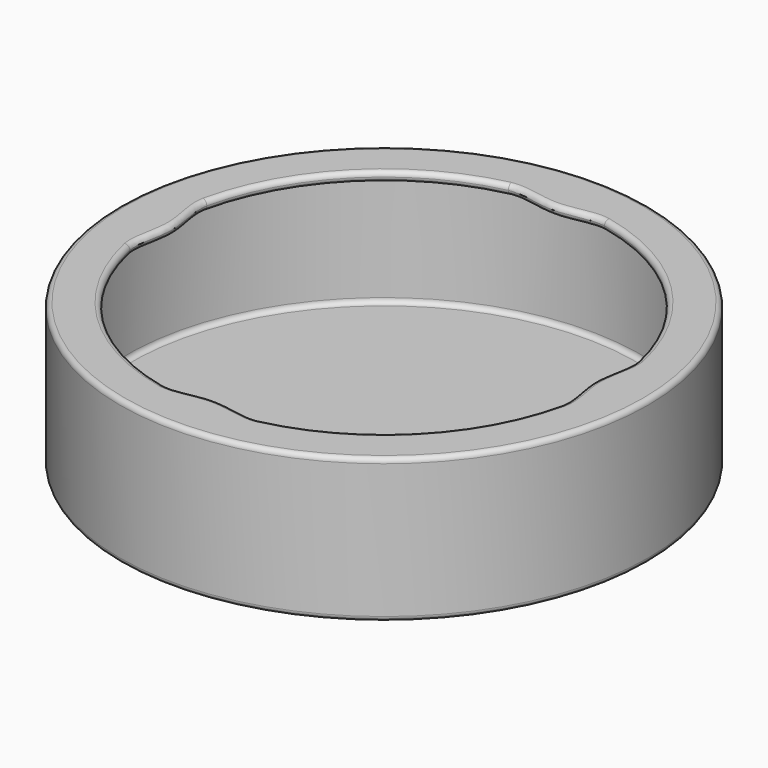
from build123d import *

# Parameters (mm, degrees)
F0_R     = 27.5
F0_R_2   = 26.75
F1_DEPTH = 1
F2_DEPTH = 15
F3_START = 14
F3_DEPTH = 1
F4_R     = 0.4999


# Not quite as in the source:
# - a fillet or chamfer is up to 0.001 mm smaller than in the source, because OpenCascade refuses the exact size


with BuildPart() as f1:
    # F0 (on Top) → F1 (new body)
    with BuildSketch(Plane.XY):
        Circle(F0_R)
        Circle(F0_R_2, mode=Mode.SUBTRACT)
        Circle(F0_R_2)
        with BuildLine():
            ThreePointArc((22.4499443206, 5), (22.8620725151, 2.5150825658), (23, 0))
            ThreePointArc((23, 0), (22.8620725151, -2.5150825658), (22.4499443206, -5))
            ThreePointArc((22.4499443206, -5), (16.2634559673, -16.2634559673), (5, -22.4499443206))
            ThreePointArc((5, -22.4499443206), (0, -23), (-5, -22.4499443206))
            ThreePointArc((-5, -22.4499443206), (-16.2634559673, -16.2634559673), (-22.4499443206, -5))
            ThreePointArc((-22.4499443206, -5), (-23, 0), (-22.4499443206, 5))
            ThreePointArc((-22.4499443206, 5), (-16.2634559673, 16.2634559673), (-5, 22.4499443206))
            ThreePointArc((-5, 22.4499443206), (0, 23), (5, 22.4499443206))
            ThreePointArc((5, 22.4499443206), (16.2634559673, 16.2634559673), (22.4499443206, 5))
        make_face(mode=Mode.SUBTRACT)
        with BuildLine():
            add(Edge.make_bspline(
                [(22.4499443206, 5), (22.7321358433, 3.5), (21.2678641567, 0), (22.7321358433, -3.5), (22.4499443206, -5)],
                knots=[0, 0, 0, 0, 0.5, 1, 1, 1, 1], degree=3))
            ThreePointArc((22.4499443206, 5), (16.2634559673, 16.2634559673), (5, 22.4499443206))
            add(Edge.make_bspline(
                [(-5, 22.4499443206), (-3.5, 22.7321358433), (0, 21.2678641567), (3.5, 22.7321358433), (5, 22.4499443206)],
                knots=[0, 0, 0, 0, 0.5, 1, 1, 1, 1], degree=3))
            ThreePointArc((-5, 22.4499443206), (-16.2634559673, 16.2634559673), (-22.4499443206, 5))
            add(Edge.make_bspline(
                [(-22.4499443206, 5), (-22.7321358433, 3.5), (-21.2678641567, 0), (-22.7321358433, -3.5), (-22.4499443206, -5)],
                knots=[0, 0, 0, 0, 0.5, 1, 1, 1, 1], degree=3))
            ThreePointArc((-22.4499443206, -5), (-16.2634559673, -16.2634559673), (-5, -22.4499443206))
            add(Edge.make_bspline(
                [(-5, -22.4499443206), (-3.5, -22.7321358433), (0, -21.2678641567), (3.5, -22.7321358433), (5, -22.4499443206)],
                knots=[0, 0, 0, 0, 0.5, 1, 1, 1, 1], degree=3))
            ThreePointArc((5, -22.4499443206), (16.2634559673, -16.2634559673), (22.4499443206, -5))
        make_face()
        with BuildLine():
            ThreePointArc((-5, -22.4499443206), (0, -23), (5, -22.4499443206))
            add(Edge.make_bspline(
                [(-5, -22.4499443206), (-3.5, -22.7321358433), (0, -21.2678641567), (3.5, -22.7321358433), (5, -22.4499443206)],
                knots=[0, 0, 0, 0, 0.5, 1, 1, 1, 1], degree=3))
        make_face()
        with BuildLine():
            add(Edge.make_bspline(
                [(-5, 22.4499443206), (-3.5, 22.7321358433), (0, 21.2678641567), (3.5, 22.7321358433), (5, 22.4499443206)],
                knots=[0, 0, 0, 0, 0.5, 1, 1, 1, 1], degree=3))
            ThreePointArc((5, 22.4499443206), (0, 23), (-5, 22.4499443206))
        make_face()
        with BuildLine():
            add(Edge.make_bspline(
                [(-22.4499443206, 5), (-22.7321358433, 3.5), (-21.2678641567, 0), (-22.7321358433, -3.5), (-22.4499443206, -5)],
                knots=[0, 0, 0, 0, 0.5, 1, 1, 1, 1], degree=3))
            ThreePointArc((-22.4499443206, 5), (-23, 0), (-22.4499443206, -5))
        make_face()
        with BuildLine():
            ThreePointArc((22.4499443206, -5), (22.8620725151, -2.5150825658), (23, 0))
            ThreePointArc((23, 0), (22.8620725151, 2.5150825658), (22.4499443206, 5))
            add(Edge.make_bspline(
                [(22.4499443206, 5), (22.7321358433, 3.5), (21.2678641567, 0), (22.7321358433, -3.5), (22.4499443206, -5)],
                knots=[0, 0, 0, 0, 0.5, 1, 1, 1, 1], degree=3))
        make_face()
    extrude(amount=F1_DEPTH)

    # F0 (on Top) → F2 (join)
    with BuildSketch(Plane.XY):
        Circle(F0_R)
        Circle(F0_R_2, mode=Mode.SUBTRACT)
    extrude(amount=F2_DEPTH)

    # F0 (on Top) → F3 (join)
    with BuildSketch(Plane.XY.offset(F3_START)):
        Circle(F0_R)
        Circle(F0_R_2, mode=Mode.SUBTRACT)
        Circle(F0_R_2)
        with BuildLine():
            ThreePointArc((22.4499443206, 5), (22.8620725151, 2.5150825658), (23, 0))
            ThreePointArc((23, 0), (22.8620725151, -2.5150825658), (22.4499443206, -5))
            ThreePointArc((22.4499443206, -5), (16.2634559673, -16.2634559673), (5, -22.4499443206))
            ThreePointArc((5, -22.4499443206), (0, -23), (-5, -22.4499443206))
            ThreePointArc((-5, -22.4499443206), (-16.2634559673, -16.2634559673), (-22.4499443206, -5))
            ThreePointArc((-22.4499443206, -5), (-23, 0), (-22.4499443206, 5))
            ThreePointArc((-22.4499443206, 5), (-16.2634559673, 16.2634559673), (-5, 22.4499443206))
            ThreePointArc((-5, 22.4499443206), (0, 23), (5, 22.4499443206))
            ThreePointArc((5, 22.4499443206), (16.2634559673, 16.2634559673), (22.4499443206, 5))
        make_face(mode=Mode.SUBTRACT)
        with BuildLine():
            add(Edge.make_bspline(
                [(-5, 22.4499443206), (-3.5, 22.7321358433), (0, 21.2678641567), (3.5, 22.7321358433), (5, 22.4499443206)],
                knots=[0, 0, 0, 0, 0.5, 1, 1, 1, 1], degree=3))
            ThreePointArc((5, 22.4499443206), (0, 23), (-5, 22.4499443206))
        make_face()
        with BuildLine():
            ThreePointArc((-5, -22.4499443206), (0, -23), (5, -22.4499443206))
            add(Edge.make_bspline(
                [(-5, -22.4499443206), (-3.5, -22.7321358433), (0, -21.2678641567), (3.5, -22.7321358433), (5, -22.4499443206)],
                knots=[0, 0, 0, 0, 0.5, 1, 1, 1, 1], degree=3))
        make_face()
        with BuildLine():
            add(Edge.make_bspline(
                [(-22.4499443206, 5), (-22.7321358433, 3.5), (-21.2678641567, 0), (-22.7321358433, -3.5), (-22.4499443206, -5)],
                knots=[0, 0, 0, 0, 0.5, 1, 1, 1, 1], degree=3))
            ThreePointArc((-22.4499443206, 5), (-23, 0), (-22.4499443206, -5))
        make_face()
        with BuildLine():
            ThreePointArc((22.4499443206, -5), (22.8620725151, -2.5150825658), (23, 0))
            ThreePointArc((23, 0), (22.8620725151, 2.5150825658), (22.4499443206, 5))
            add(Edge.make_bspline(
                [(22.4499443206, 5), (22.7321358433, 3.5), (21.2678641567, 0), (22.7321358433, -3.5), (22.4499443206, -5)],
                knots=[0, 0, 0, 0, 0.5, 1, 1, 1, 1], degree=3))
        make_face()
    extrude(amount=F3_DEPTH)

    # F4 (radius 0.5 in the source; OpenCascade refuses exactly that, so slightly less here)
    f4_edges = [f1.edges().sort_by_distance(p)[0] for p in [
        (-26.75, 0, 1),
        (-27.5, 0, 0),
        (-27.5, 0, 15),
        (-22, 0, 14),
        (-22, 0, 15),
        (-16.263456, -16.263456, 15),
        (-16.263456, -16.263456, 14),
        (16.263456, -16.263456, 15),
        (0, -22, 15),
        (0, -22, 14),
        (16.263456, -16.263456, 14),
        (22, 0, 15),
        (22, 0, 14),
        (-16.263456, 16.263456, 15),
        (-16.263456, 16.263456, 14),
        (0, 22, 15),
        (0, 22, 14),
        (16.263456, 16.263456, 14),
        (16.263456, 16.263456, 15),
        (-26.75, 0, 14),
    ]]
    fillet(f4_edges, radius=F4_R)


solid = f1.part
